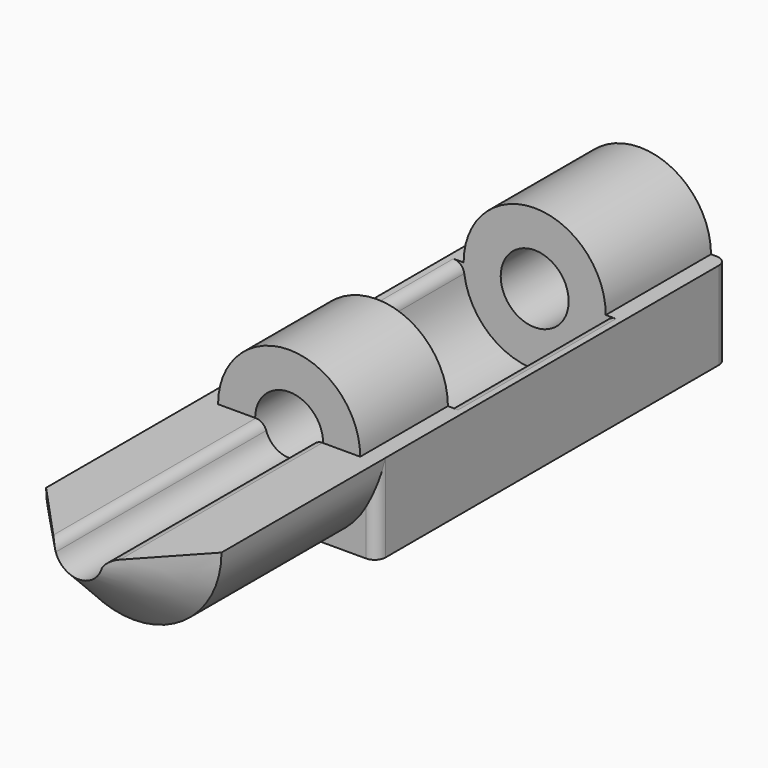
from build123d import *

# Parameters (mm, degrees)
F0_W     = 0.7586409766
F0_H     = 4.9999998882
F0_H_2   = 9
F0_H_3   = 6.0000001118
F1_ANGLE = 180
F0_W_2   = 1.6913590234
F4_DEPTH = 20
F5_R     = 0.5


with BuildPart() as f1:
    # F0 (on Top) → F1 (revolve)
    with BuildSketch(Plane.XY):
        Polygon((-4, -8.8572846726), (-1.1, -12), (-1.1, 0), (-1.55, 0), (-3.2413590234, 0), (-4, 0), align=None)
        with Locations((-3.6206795117, 2.4999999441)):
            Rectangle(F0_W, F0_H)
        with Locations((-3.6206795117, 9.4999998882)):
            Rectangle(F0_W, F0_H_2)
        with Locations((-3.6206795117, 16.9999999441)):
            Rectangle(F0_W, F0_H_3)
    revolve(axis=Axis((0, 4.4247480631, 0), (0, -1, 0)), revolution_arc=F1_ANGLE)

    # F0 (on Top) → F2 (revolve)
    with BuildSketch(Plane.XY):
        with Locations((-2.3956795117, 2.4999999441)):
            Rectangle(F0_W_2, F0_H)
        with Locations((-2.3956795117, 16.9999999441)):
            Rectangle(F0_W_2, F0_H_3)
    revolve(axis=Axis((0, 4.4247480631, 0), (0, -1, 0)))

    # F3 (on face) → F4 (join)
    with BuildSketch(Plane(origin=(0, 20, 0), x_dir=(-1, 0, 0), z_dir=(0, 1, 0))):
        with BuildLine():
            ThreePointArc((0, -4), (-2.8284271247, -2.8284271247), (-4, 0))
            Line((-4, 0), (-4, -4))
            Line((-4, -4), (0, -4))
        make_face()
        with BuildLine():
            ThreePointArc((4, 0), (2.8284271247, -2.8284271247), (0, -4))
            Line((0, -4), (4, -4))
            Line((4, -4), (4, 0))
        make_face()
    extrude(amount=-F4_DEPTH)

    # F5
    f5_edges = [f1.edges().sort_by_distance(p)[0] for p in [
        (1.1, -6, 0),
        (-1.1, -6, 0),
        (1.55, 5, 0),
        (1.55, 20, 0),
        (3.241359, 9.5, 0),
        (-3.241359, 9.5, 0),
        (4, 20, -2),
        (-4, 20, -2),
        (4, 0, -2),
        (-4, 0, -2),
    ]]
    fillet(f5_edges, radius=F5_R)


solid = f1.part
